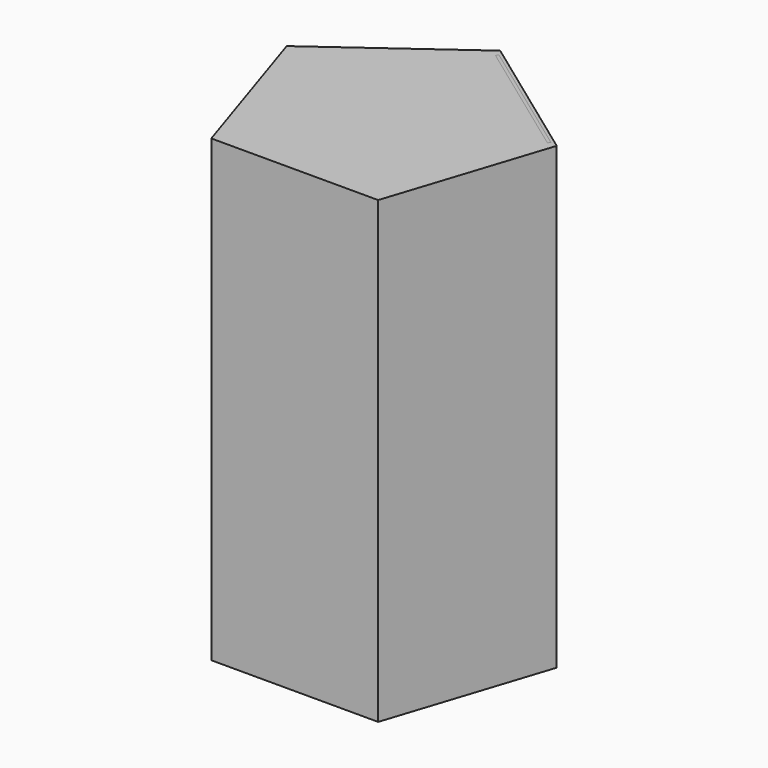
from build123d import *

# Parameters (mm, degrees)
F4_DEPTH = 161.803
F5_DEPTH = 25
F6_START = 131.803
F6_DEPTH = 5
F7_DEPTH = 161.803


with BuildPart() as f4:
    # F3 (on Top) → F4 (new body)
    with BuildSketch(Plane.XY):
        Polygon((2.3974051677, 48.2581831888), (0, 50), (-47.5528258148, 15.4508497187), (-29.3892626146, -40.4508497187), (29.3892626146, -40.4508497187), (47.5528258148, 15.4508497187), (45.1554206471, 17.1926665299), (44.5676353948, 16.3836495356), (45.0530455914, 16.0309783842), (44.4652603391, 15.2219613898), (43.9798501425, 15.5746325412), (43.7288358726, 15.2291410384), (44.6996562659, 14.5237987356), (27.6259068577, -38.0237987356), (-27.6259068577, -38.0237987356), (-44.6996562659, 14.5237987356), (0, 47), (0.9708203932, 46.2946576972), (1.2218346631, 46.6401492001), (0.7364244665, 46.9928203514), (1.3242097188, 47.8018373458), (1.8096199154, 47.4491661944), align=None)
    extrude(amount=F4_DEPTH)

    # F3 (on Top) → F5 (join)
    with BuildSketch(Plane.XY):
        Polygon((2.3974051677, 48.2581831888), (0, 50), (-47.5528258148, 15.4508497187), (-29.3892626146, -40.4508497187), (29.3892626146, -40.4508497187), (47.5528258148, 15.4508497187), (45.1554206471, 17.1926665299), (44.5676353948, 16.3836495356), (45.0530455914, 16.0309783842), (44.4652603391, 15.2219613898), (43.9798501425, 15.5746325412), (43.7288358726, 15.2291410384), (44.6996562659, 14.5237987356), (27.6259068577, -38.0237987356), (-27.6259068577, -38.0237987356), (-44.6996562659, 14.5237987356), (0, 47), (0.9708203932, 46.2946576972), (1.2218346631, 46.6401492001), (0.7364244665, 46.9928203514), (1.3242097188, 47.8018373458), (1.8096199154, 47.4491661944), align=None)
        Polygon((45.1554206471, 17.1926665299), (2.3974051677, 48.2581831888), (1.8096199154, 47.4491661944), (44.5676353948, 16.3836495356), align=None)
        Polygon((43.7288358726, 15.2291410384), (0.9708203932, 46.2946576972), (0, 47), (-44.6996562659, 14.5237987356), (-27.6259068577, -38.0237987356), (27.6259068577, -38.0237987356), (44.6996562659, 14.5237987356), align=None)
        Polygon((44.5676353948, 16.3836495356), (1.8096199154, 47.4491661944), (1.3242097188, 47.8018373458), (0.7364244665, 46.9928203514), (1.2218346631, 46.6401492001), (43.9798501425, 15.5746325412), (44.4652603391, 15.2219613898), (45.0530455914, 16.0309783842), align=None)
        Polygon((43.9798501425, 15.5746325412), (1.2218346631, 46.6401492001), (0.9708203932, 46.2946576972), (43.7288358726, 15.2291410384), align=None)
    extrude(amount=F5_DEPTH)

    # F5_face (on face) → F6 (join)
    with BuildSketch(Plane(origin=(0.5548214396, 0.7636461986, 25), x_dir=(1, 0, 0), z_dir=(0, 0, 1)).offset(F6_START)):
        Polygon((44.0128139551, 15.6200033369), (44.6005992074, 16.4290203313), (1.8425837281, 47.4945369902), (1.2547984758, 46.6855199958), (0.7693882791, 47.0381911472), (0.1816030268, 46.2291741528), (0.6670132235, 45.8765030014), (0.4159989536, 45.5310114986), (-0.5548214396, 46.2363538014), (-45.2544777055, 13.760152537), (-28.1807282974, -38.7874449342), (27.0710854181, -38.7874449342), (44.1448348262, 13.760152537), (43.174014433, 14.4654948398), (43.4250287028, 14.8109863426), (43.9104388995, 14.4583151912), (44.4982241518, 15.2673321856), align=None)
    extrude(amount=F6_DEPTH)


with BuildPart() as f7:
    # F3 (on Top) → F7 (new body)
    with BuildSketch(Plane.XY):
        Polygon((44.5676353948, 16.3836495356), (1.8096199154, 47.4491661944), (1.3242097188, 47.8018373458), (0.7364244665, 46.9928203514), (1.2218346631, 46.6401492001), (43.9798501425, 15.5746325412), (44.4652603391, 15.2219613898), (45.0530455914, 16.0309783842), align=None)
    extrude(amount=F7_DEPTH)


solid = Compound([f4.part, f7.part])
